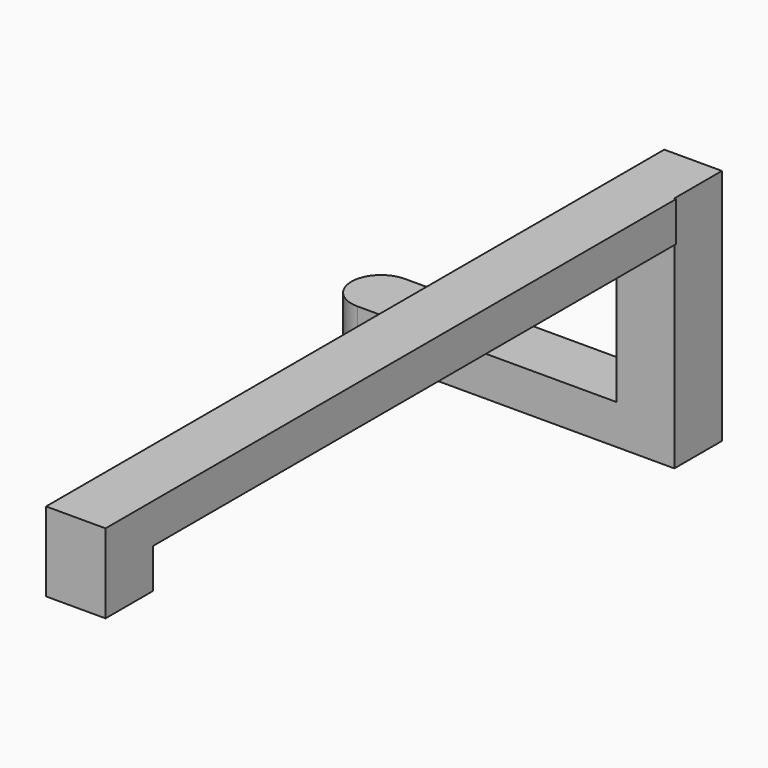
from build123d import *

# Parameters (mm, degrees)
F0_W     = 18.4755190939
F0_H     = 19.05
F1_DEPTH = 12.7
F2_DEPTH = 76.2
F4_DEPTH = 12.7
F3_W     = 19.05
F3_H     = 19.05
F5_DEPTH = 25.4


# Not quite as in the source:
# - a feature names something its author has since deleted; it is built from what else it names


with BuildPart() as f1:
    # F0 (on Top) → F1 (new body)
    with BuildSketch(Plane.XY):
        with BuildLine():
            Line((34.1462217655, 9.525), (-48.9782591407, 9.525))
            ThreePointArc((-48.9782591407, 9.525), (-58.5032591407, 0), (-48.9782591407, -9.525))
            Line((-48.9782591407, -9.525), (34.1462217655, -9.525))
            Line((34.1462217655, -9.525), (34.1462217655, 9.525))
        make_face()
        with Locations((43.3839813124, 0)):
            Rectangle(F0_W, F0_H)
    extrude(amount=F1_DEPTH)

    # F0 (on Top) → F2 (join)
    with BuildSketch(Plane.XY):
        with Locations((43.3839813124, 0)):
            Rectangle(F0_W, F0_H)
    extrude(amount=F2_DEPTH)

    # F3 (on face) → F4 (join)
    with BuildSketch(Plane.XY.offset(76.2)):
        Polygon((52.6217408593, -9.525), (34.1462217655, -9.525), (34.1462217655, -219.075), (53.1962217655, -219.075), (53.1962217655, -9.525), align=None)
    extrude(amount=-F4_DEPTH)

    # F3 (on face) → F5 (join)
    with BuildSketch(Plane.XY.offset(76.2)):
        with Locations((43.6712217655, -228.6)):
            Rectangle(F3_W, F3_H)
    extrude(amount=-F5_DEPTH)


with BuildPart() as f6_1:
    # F6: copy of F1
    add(f1.part)


solid = f1.part
